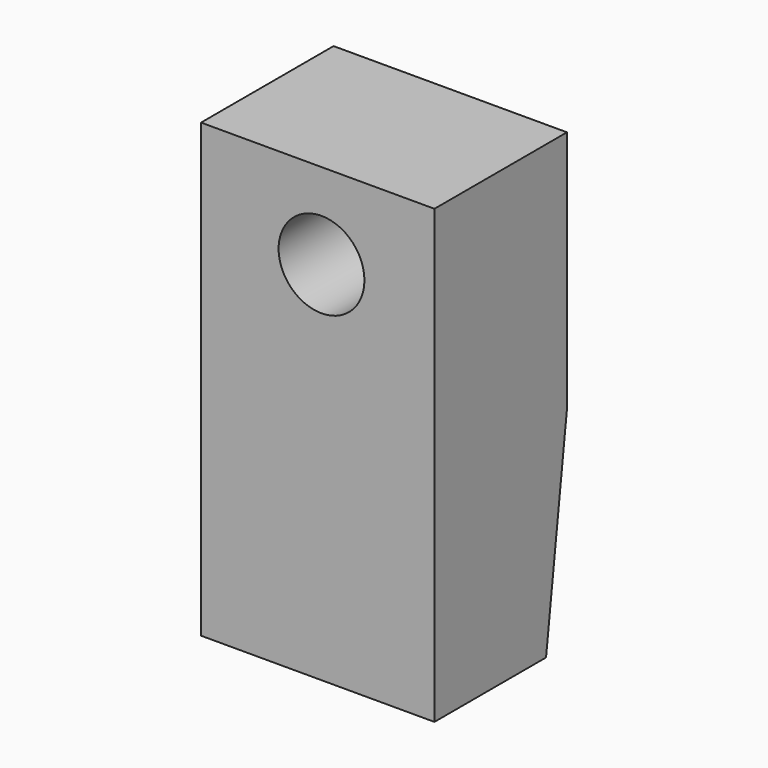
from build123d import *

# Parameters (mm, degrees)
F0_W     = 7.874
F0_H     = 15.24
F0_R     = 1.4478
F1_DEPTH = 5.588
F2_R     = 2.794
F3_DEPTH = 1.27
F5_DEPTH = 25.4


# Not quite as in the source:
# - a feature names something its author has since deleted; it is built from what else it names


with BuildPart() as f1:
    # F0 (on Front) → F1 (new body)
    with BuildSketch(Plane.XZ):
        with Locations((-104.3903227065, 34.7791743618)):
            Rectangle(F0_W, F0_H)
        with Locations((-104.2633227065, 39.5035743618)):
            Circle(F0_R, mode=Mode.SUBTRACT)
    extrude(amount=F1_DEPTH)

    # F2 (on face) → F3 (cut)
    with BuildSketch(Plane(origin=(0, 0, 0), x_dir=(-1, 0, 0), z_dir=(0, 1, 0))):
        with Locations((104.2633227065, 39.5035743618)):
            Circle(F2_R)
    extrude(amount=-F3_DEPTH, mode=Mode.SUBTRACT)

    # F4 (on face) → F5 (cut)
    with BuildSketch(Plane.YZ.offset(-100.4533227065)):
        Polygon((0, 34.1825485229), (-0.8814302273, 27.1591743618), (0, 27.1591743618), align=None)
    extrude(amount=-F5_DEPTH, mode=Mode.SUBTRACT)


solid = f1.part
